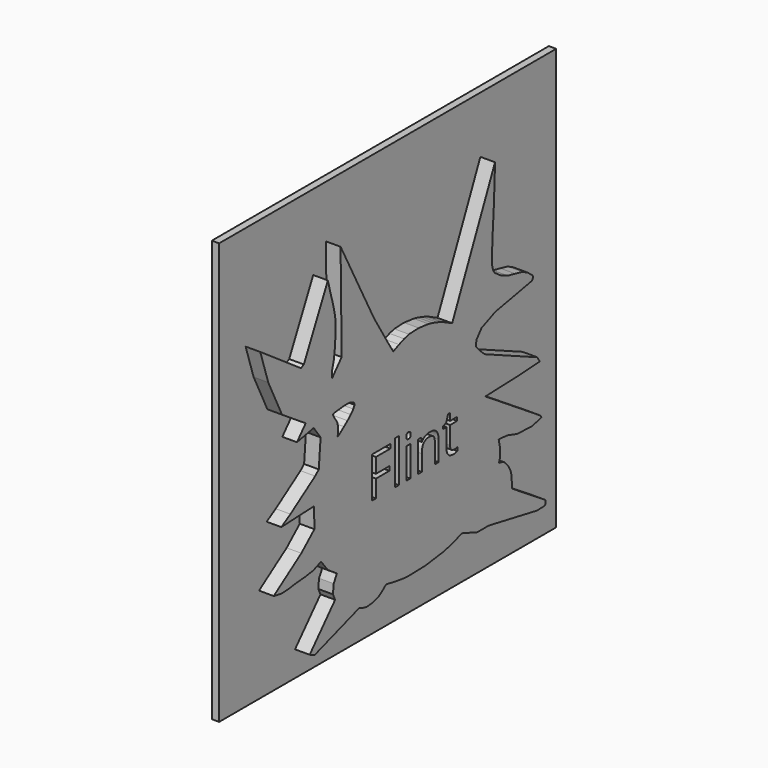
from build123d import *

# Parameters (mm, degrees)
F1_DEPTH     = 6.35
F2_W         = 146.05
F2_H         = 146.05
F3_DEPTH     = 1.27
F4_TEXT_SIZE = 19.7550320687
F5_DEPTH     = 25.4


# Not quite as in the source:
# - Text() gives the source's letters only with a copy of the font that has no kerning and outlines rounded to 1/6400 em; it was checked with that copy


with BuildPart() as f1:
    # F0 (on Right) → F1 (new body, symmetric)
    with BuildSketch(Plane.YZ):
        Polygon((-26.4927588, 59.0158586), (-27.0093948, 60.0039186), (-26.5367008, 26.1426706), (-30.7894228, 21.2618066), (-30.7894228, 23.4667806), (-30.6751228, 23.8607346), (-30.4035968, 24.8185686), (-30.0909228, 26.0050026), (-29.8440348, 27.0880586), (-29.5300908, 29.7657266), (-29.1800788, 34.1782146), (-29.2143688, 38.5851146), (-29.6581068, 41.1853126), (-30.3484788, 44.0242706), (-30.9839868, 46.3102706), (-31.2621168, 47.2475306), (-32.5217028, 51.9711686), (-42.9161448, 30.5523646), (-44.1757308, 29.9226986), (-61.8146592, 42.0494206), (-58.350277, 31.3407806), (-52.3654782, 19.0570866), (-42.1292528, 12.2836686), (-45.9080108, 8.0327246), (-38.6634228, 9.4490286), (-35.6720648, 5.3550566), (-36.4587028, -4.0939974), (-38.0337568, -5.5120794), (-48.7439208, -12.7564134), (-52.6810224, -15.1183594), (-46.0665068, -14.8044154), (-38.5064508, -14.4886934), (-38.3494788, -21.5758014), (-44.0187588, -26.6154154), (-55.9883056, -34.8051374), (-55.5955708, -34.8975934), (-54.6364668, -35.1028254), (-53.4486104, -35.3177094), (-52.3654782, -35.4348034), (-49.2910368, -35.2295714), (-46.2234788, -34.8051374), (-42.6598588, -34.5295474), (-39.1361168, -34.0184994), (-38.0408688, -33.6641694), (-36.8541808, -33.1914754), (-35.9047288, -32.7779634), (-35.5148388, -32.6001634), (-32.5217028, -36.3801914), (-28.5847028, -39.0578594), (-30.0027848, -41.5767774), (-30.3167288, -44.7271394), (-29.3713408, -46.7746334), (-40.3957028, -59.0586322), (-38.1907288, -60.0039186), (-18.9784228, -53.5465274), (-18.6228228, -53.6885134), (-17.7546508, -54.003956), (-16.6713408, -54.3264344), (-15.6713428, -54.491763), (-13.0127248, -54.2368486), (-10.4729788, -53.3893014), (-9.9949508, -53.1317454), (-9.4783148, -52.7898614), (-8.9517728, -52.4027654), (-8.4501228, -52.0044934), (-8.0051148, -51.6311134), (-7.6479908, -51.3194554), (-7.4099928, -51.1058414), (-7.3226168, -51.0273554), (-7.0485508, -51.0824734), (-6.2946788, -51.2328414), (-5.1732688, -51.4462014), (-3.7925248, -51.6943594), (-2.2629368, -51.9478514), (-0.6932168, -52.1767054), (0.8058912, -52.3517114), (2.1264372, -52.4441674), (9.8736912, -52.2318234), (17.5604932, -51.1845814), (19.9719692, -50.6001274), (22.6041712, -49.8119654), (24.7217692, -49.1187994), (25.5914652, -48.8226354), (32.2061332, -51.1845814), (36.9315492, -51.1845814), (38.0339092, -51.3415534), (58.1916032, -55.121556), (61.6576872, -54.964457), (61.8146592, -53.3893014), (47.1672412, -43.9402474), (47.1730832, -43.7733694), (47.1824812, -43.3215034), (47.1852752, -42.6514514), (47.1687652, -41.8330634), (47.1232992, -40.9318714), (47.0364312, -40.0184874), (46.8974932, -39.1612374), (46.6963252, -38.4281934), (45.6229212, -36.3390434), (44.0186572, -34.6481654), (43.3668932, -34.3156794), (42.5868592, -34.0677754), (41.9295072, -33.9120734), (41.6551872, -33.8597494), (42.1278812, -32.1274694), (42.1278812, -29.6085514), (41.4982152, -26.6154154), (45.2782432, -26.9311374), (49.3722152, -28.1904694), (55.9868832, -28.5061914), (60.0826332, -27.4038314), (59.4527132, -26.6154154), (39.6089632, -13.7018014), (35.6719632, -11.1813594), (49.2152432, -10.7086654), (59.2939632, -10.0789994), (58.1916032, -8.3467194), (35.9861612, 1.5750286), (35.3562412, 1.8889726), (33.4672432, 3.6230306), (31.5762132, 5.6690006), (31.8919352, 7.7170026), (34.0969092, 10.3946706), (40.0816572, 12.9133346), (50.1606312, 14.8043646), (55.8299112, 15.9067246), (55.9744372, 16.0484566), (56.2431692, 16.4149786), (56.3836312, 16.9224706), (56.1456332, 17.4817786), (54.1004252, 19.1287146), (51.7356852, 20.3164186), (48.5949752, 21.0494626), (45.4352152, 21.7329766), (42.4255692, 23.0339646), (39.7659352, 24.8830846), (39.1969752, 25.7845306), (38.8055612, 26.9351506), (38.5782312, 27.9272746), (38.5066032, 28.3473906), (38.8205472, 36.0644186), (39.4502132, 46.3021426), (39.9231612, 58.5858366), (21.3405212, 17.0090846), (16.9308272, 19.2140586), (16.3006532, 19.4388486), (14.7657312, 19.9565006), (12.8559052, 20.5368906), (11.1027972, 20.9460846), (6.8500752, 21.4464646), (2.5991312, 21.2618066), (0.5361432, 20.7063086), (-1.6797528, 19.8589646), (-3.4506408, 19.0817246), (-4.1742868, 18.7413646), (-6.3790068, 22.2056706), (-12.5209808, 32.2861686), (-12.7455168, 32.7159366), (-13.4041388, 33.9767926), (-14.4777968, 36.0316526), (-15.9466788, 38.8414006), (-17.7917348, 42.3704766), (-19.9913748, 46.5790026), (-22.5268028, 51.4296406), (-25.3779528, 56.8840366), (-25.5339088, 57.1817246), (-25.6273808, 57.3610486), (-25.6974848, 57.4946526), (-25.7818128, 57.6544186), (-25.9169408, 57.9134986), (-26.1412228, 58.3435206), align=None)
        Polygon((-27.8872188, 2.7810206), (-28.2689808, 2.5206706), (-28.2346908, 2.9545026), (-28.1767788, 4.0058086), (-28.1656028, 5.2996846), (-28.2689808, 6.4576706), (-28.4716728, 7.0223126), (-28.8272728, 7.6468986), (-29.2570408, 8.2915506), (-29.6870628, 8.9146126), (-30.0370748, 9.4779846), (-30.2313848, 9.9397566), (-30.1930308, 10.2580186), (-29.8440348, 10.3946706), (-27.6558248, 10.6316526), (-25.2413008, 10.8823506), (-22.9621588, 10.8109766), (-21.1833968, 10.0789486), (-20.9448908, 9.3029786), (-21.4920068, 8.2338926), (-22.5930968, 6.9961506), (-24.0165128, 5.7093866), (-25.5280668, 4.4978066), (-26.8966188, 3.4807906), align=None, mode=Mode.SUBTRACT)
    extrude(amount=F1_DEPTH, both=True)

    # F2 (on Right) → F3 (join, symmetric)
    with BuildSketch(Plane.YZ):
        with Locations((-0.2564415336, 5.1801328065)):
            Rectangle(F2_W, F2_H)
    extrude(amount=F3_DEPTH, both=True)

    # F4 (on Right) → F5 (cut, symmetric)
    with BuildSketch(Plane.YZ):
        with Locations((-15.2761780191, -23.0124555528)):
            Text('Flint', F4_TEXT_SIZE, font='Open Sans', text_align=(TextAlign.LEFT, TextAlign.BOTTOM))
    extrude(amount=F5_DEPTH, both=True, mode=Mode.SUBTRACT)


solid = f1.part
